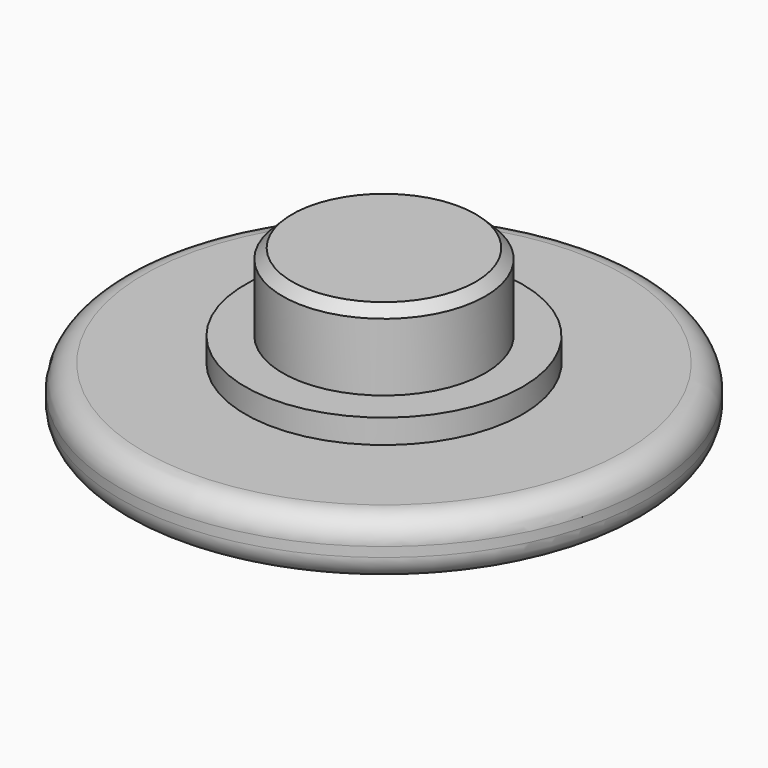
from build123d import *

# Parameters (mm, degrees)
F0_R     = 10.95
F1_DEPTH = 2.4
F2_R     = 4.2
F3_DEPTH = 4.2
F4_R     = 1
F5_R     = 5.75
F5_R_2   = 4.2
F6_DEPTH = 1
F7_R     = 1
F8_R     = 8
F9_DEPTH = 1
F11_SIZE = 0.4
F12_R    = 6


# Not quite as in the source:
# - a fillet or chamfer that OpenCascade refuses, or shapes differently, is made with other operations: its cross-section is extruded or revolved along the edge and cut away or added


with BuildPart() as f1:
    # F0 (on Top) → F1 (new body)
    with BuildSketch(Plane.XY):
        Circle(F0_R)
    extrude(amount=F1_DEPTH)

    # F2 (on face) → F3 (join)
    with BuildSketch(Plane.XY.offset(2.4)):
        Circle(F2_R)
    extrude(amount=F3_DEPTH)

    # F4
    f4_edges = [f1.edges().sort_by_distance(p)[0] for p in [
        (-10.95, 0, 2.4),
    ]]
    fillet(f4_edges, radius=F4_R)

    # F5 (on face) → F6 (join)
    with BuildSketch(Plane.XY.offset(2.4)):
        Circle(F5_R)
        Circle(F5_R_2, mode=Mode.SUBTRACT)
    extrude(amount=F6_DEPTH)

    # F7
    f7_edges = [f1.edges().sort_by_distance(p)[0] for p in [
        (-10.95, 0, 0),
    ]]
    fillet(f7_edges, radius=F7_R)

    # F8 (on face) → F9 (cut)
    with BuildSketch(Plane(origin=(0, 0, 0), x_dir=(1, 0, 0), z_dir=(0, 0, -1))):
        Circle(F8_R)
    extrude(amount=-F9_DEPTH, mode=Mode.SUBTRACT)

    # F10: fillet of radius 11 on 1 edges, made by hand

    # F10_s1 → F10_t2 (revolve)
    with BuildSketch(Plane.XZ):
        with BuildLine():
            ThreePointArc((8, 0), (5.762632185, 0.7470926301), (3.417424305, 1))
            Line((3.417424305, 1), (8, 1))
            Line((8, 1), (8, 0))
        make_face()
    revolve(axis=Axis((0, 0, 1), (0, 0, -1)))

    # F11
    f11_edges = [f1.edges().sort_by_distance(p)[0] for p in [
        (-4.2, 0, 6.6),
    ]]
    chamfer(f11_edges, length=F11_SIZE)

    # F12
    f12_edges = [f1.edges().sort_by_distance(p)[0] for p in [
        (-8, 0, 0),
    ]]
    fillet(f12_edges, radius=F12_R)


solid = f1.part
